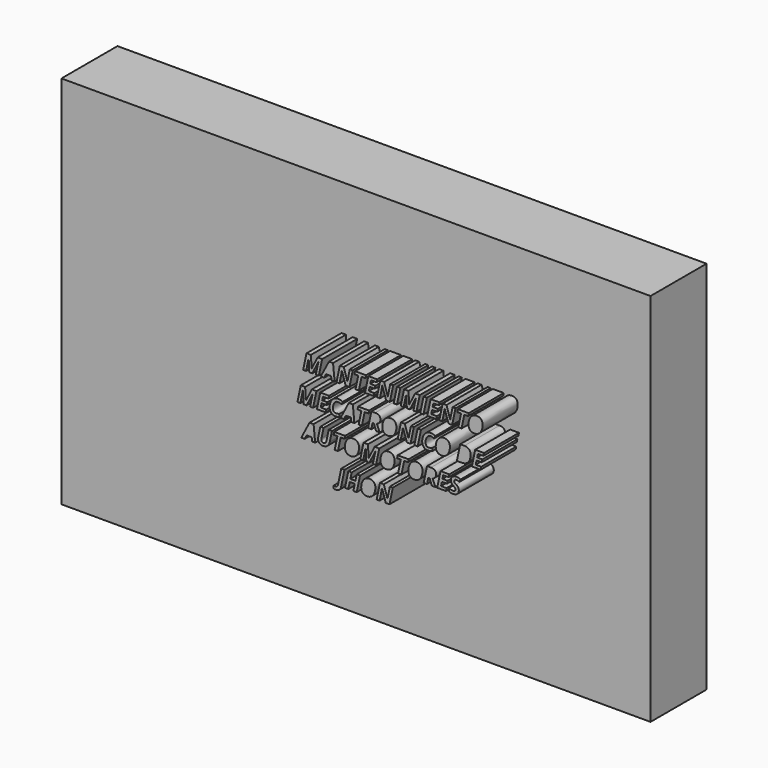
from build123d import *

# Parameters (mm, degrees)
F0_W         = 143.1818306446
F0_H         = 107.0454642177
F1_DEPTH     = 20
F3_DEPTH     = 25
F2_TEXT_SIZE = 6.3131304665
F4_DEPTH     = 12.5


# Not quite as in the source:
# - Text() gives the source's letters only with a copy of the font that has no kerning and outlines rounded to 1/6400 em; it was checked with that copy


with BuildPart() as f1:
    # F0 (on Front) → F1 (new body)
    with BuildSketch(Plane.XZ):
        Rectangle(F0_W, F0_H)
    extrude(amount=F1_DEPTH)

    # F3 (add): a face of the model
    f3_faces = [f1.faces().sort_by_distance(p)[0] for p in [
        (-71.5909153223, -10, 0),
    ]]
    extrude(f3_faces, amount=F3_DEPTH)

    # F2 (on face) → F4 (join, symmetric)
    with BuildSketch(Plane.XZ.offset(20)):
        with Locations((-7.8935887165, -14.7348443667)):
            Text('JHON', F2_TEXT_SIZE, font='Open Sans', font_style=FontStyle.BOLDITALIC, text_align=(TextAlign.LEFT, TextAlign.BOTTOM))
        with Locations((-17.7361536844, -6.1489869323)):
            Text('AUTOMOTORES', F2_TEXT_SIZE, font='Open Sans', font_style=FontStyle.BOLDITALIC, text_align=(TextAlign.LEFT, TextAlign.BOTTOM))
        with BuildLine():
            add(Edge.make_bspline(
                [(7.8744410502, 5.9801149764), (7.6741964432, 6.2188302222), (7.3102050147, 6.2188302222)],
                knots=[0, 0, 0, 1, 1, 1], degree=2))
            add(Edge.make_bspline(
                [(7.3102050147, 6.2188302222), (6.9373357465, 6.2188302222), (6.6261181431, 5.9372054178)],
                knots=[0, 0, 0, 1, 1, 1], degree=2))
            add(Edge.make_bspline(
                [(6.6261181431, 5.9372054178), (6.3149005396, 5.6555806134), (6.1373437452, 5.1623672957)],
                knots=[0, 0, 0, 1, 1, 1], degree=2))
            add(Edge.make_bspline(
                [(6.1373437452, 5.1623672957), (5.9597869509, 4.669153978), (5.9597869509, 4.0920943963)],
                knots=[0, 0, 0, 1, 1, 1], degree=2))
            add(Edge.make_bspline(
                [(5.9597869509, 4.0920943963), (5.9597869509, 3.6393245706), (6.164963691, 3.4080075246)],
                knots=[0, 0, 0, 1, 1, 1], degree=2))
            add(Edge.make_bspline(
                [(6.164963691, 3.4080075246), (6.3701404312, 3.1766904786), (6.7430096994, 3.1766904786)],
                knots=[0, 0, 0, 1, 1, 1], degree=2))
            add(Edge.make_bspline(
                [(6.7430096994, 3.1766904786), (7.1158789675, 3.1766904786), (7.4226576512, 3.4449985235)],
                knots=[0, 0, 0, 1, 1, 1], degree=2))
            add(Edge.make_bspline(
                [(7.4226576512, 3.4449985235), (7.7294363348, 3.7133065683), (7.902060996, 4.2035606061)],
                knots=[0, 0, 0, 1, 1, 1], degree=2))
            add(Edge.make_bspline(
                [(7.902060996, 4.2035606061), (8.0746856571, 4.6938146439), (8.0746856571, 5.3034263045)],
                knots=[0, 0, 0, 1, 1, 1], degree=2))
            add(Edge.make_bspline(
                [(8.0746856571, 5.3034263045), (8.0746856571, 5.7413997306), (7.8744410502, 5.9801149764)],
                knots=[0, 0, 0, 1, 1, 1], degree=2))
        make_face()
        with BuildLine():
            add(Edge.make_bspline(
                [(32.4936770161, 14.5659724108), (32.2934324092, 14.8046876566), (31.9294409807, 14.8046876566)],
                knots=[0, 0, 0, 1, 1, 1], degree=2))
            add(Edge.make_bspline(
                [(31.9294409807, 14.8046876566), (31.5565717125, 14.8046876566), (31.2453541091, 14.5230628522)],
                knots=[0, 0, 0, 1, 1, 1], degree=2))
            add(Edge.make_bspline(
                [(31.2453541091, 14.5230628522), (30.9341365056, 14.2414380478), (30.7565797112, 13.7482247301)],
                knots=[0, 0, 0, 1, 1, 1], degree=2))
            add(Edge.make_bspline(
                [(30.7565797112, 13.7482247301), (30.5790229169, 13.2550114124), (30.5790229169, 12.6779518307)],
                knots=[0, 0, 0, 1, 1, 1], degree=2))
            add(Edge.make_bspline(
                [(30.5790229169, 12.6779518307), (30.5790229169, 12.225182005), (30.784199657, 11.993864959)],
                knots=[0, 0, 0, 1, 1, 1], degree=2))
            add(Edge.make_bspline(
                [(30.784199657, 11.993864959), (30.9893763972, 11.762547913), (31.3622456654, 11.762547913)],
                knots=[0, 0, 0, 1, 1, 1], degree=2))
            add(Edge.make_bspline(
                [(31.3622456654, 11.762547913), (31.7351149335, 11.762547913), (32.0418936171, 12.0308559579)],
                knots=[0, 0, 0, 1, 1, 1], degree=2))
            add(Edge.make_bspline(
                [(32.0418936171, 12.0308559579), (32.3486723007, 12.2991640027), (32.5212969619, 12.7894180405)],
                knots=[0, 0, 0, 1, 1, 1], degree=2))
            add(Edge.make_bspline(
                [(32.5212969619, 12.7894180405), (32.6939216231, 13.2796720783), (32.6939216231, 13.8892837389)],
                knots=[0, 0, 0, 1, 1, 1], degree=2))
            add(Edge.make_bspline(
                [(32.6939216231, 13.8892837389), (32.6939216231, 14.3272571651), (32.4936770161, 14.5659724108)],
                knots=[0, 0, 0, 1, 1, 1], degree=2))
        make_face()
        with BuildLine():
            add(Edge.make_bspline(
                [(15.3160435875, -2.605742458), (15.1157989805, -2.3670272122), (14.7518075521, -2.3670272122)],
                knots=[0, 0, 0, 1, 1, 1], degree=2))
            add(Edge.make_bspline(
                [(14.7518075521, -2.3670272122), (14.3789382839, -2.3670272122), (14.0677206804, -2.6486520166)],
                knots=[0, 0, 0, 1, 1, 1], degree=2))
            add(Edge.make_bspline(
                [(14.0677206804, -2.6486520166), (13.756503077, -2.930276821), (13.5789462826, -3.4234901387)],
                knots=[0, 0, 0, 1, 1, 1], degree=2))
            add(Edge.make_bspline(
                [(13.5789462826, -3.4234901387), (13.4013894882, -3.9167034564), (13.4013894882, -4.4937630381)],
                knots=[0, 0, 0, 1, 1, 1], degree=2))
            add(Edge.make_bspline(
                [(13.4013894882, -4.4937630381), (13.4013894882, -4.9465328638), (13.6065662284, -5.1778499098)],
                knots=[0, 0, 0, 1, 1, 1], degree=2))
            add(Edge.make_bspline(
                [(13.6065662284, -5.1778499098), (13.8117429686, -5.4091669558), (14.1846122367, -5.4091669558)],
                knots=[0, 0, 0, 1, 1, 1], degree=2))
            add(Edge.make_bspline(
                [(14.1846122367, -5.4091669558), (14.5574815049, -5.4091669558), (14.8642601885, -5.1408589109)],
                knots=[0, 0, 0, 1, 1, 1], degree=2))
            add(Edge.make_bspline(
                [(14.8642601885, -5.1408589109), (15.1710388721, -4.8725508661), (15.3436635333, -4.3822968283)],
                knots=[0, 0, 0, 1, 1, 1], degree=2))
            add(Edge.make_bspline(
                [(15.3436635333, -4.3822968283), (15.5162881945, -3.8920427905), (15.5162881945, -3.2824311299)],
                knots=[0, 0, 0, 1, 1, 1], degree=2))
            add(Edge.make_bspline(
                [(15.5162881945, -3.2824311299), (15.5162881945, -2.8444577038), (15.3160435875, -2.605742458)],
                knots=[0, 0, 0, 1, 1, 1], degree=2))
        make_face()
        with BuildLine():
            add(Edge.make_bspline(
                [(7.3565670666, -2.605742458), (7.1563224596, -2.3670272122), (6.7923310311, -2.3670272122)],
                knots=[0, 0, 0, 1, 1, 1], degree=2))
            add(Edge.make_bspline(
                [(6.7923310311, -2.3670272122), (6.419461763, -2.3670272122), (6.1082441595, -2.6486520166)],
                knots=[0, 0, 0, 1, 1, 1], degree=2))
            add(Edge.make_bspline(
                [(6.1082441595, -2.6486520166), (5.797026556, -2.930276821), (5.6194697617, -3.4234901387)],
                knots=[0, 0, 0, 1, 1, 1], degree=2))
            add(Edge.make_bspline(
                [(5.6194697617, -3.4234901387), (5.4419129673, -3.9167034564), (5.4419129673, -4.4937630381)],
                knots=[0, 0, 0, 1, 1, 1], degree=2))
            add(Edge.make_bspline(
                [(5.4419129673, -4.4937630381), (5.4419129673, -4.9465328638), (5.6470897075, -5.1778499098)],
                knots=[0, 0, 0, 1, 1, 1], degree=2))
            add(Edge.make_bspline(
                [(5.6470897075, -5.1778499098), (5.8522664476, -5.4091669558), (6.2251357158, -5.4091669558)],
                knots=[0, 0, 0, 1, 1, 1], degree=2))
            add(Edge.make_bspline(
                [(6.2251357158, -5.4091669558), (6.598004984, -5.4091669558), (6.9047836676, -5.1408589109)],
                knots=[0, 0, 0, 1, 1, 1], degree=2))
            add(Edge.make_bspline(
                [(6.9047836676, -5.1408589109), (7.2115623512, -4.8725508661), (7.3841870124, -4.3822968283)],
                knots=[0, 0, 0, 1, 1, 1], degree=2))
            add(Edge.make_bspline(
                [(7.3841870124, -4.3822968283), (7.5568116736, -3.8920427905), (7.5568116736, -3.2824311299)],
                knots=[0, 0, 0, 1, 1, 1], degree=2))
            add(Edge.make_bspline(
                [(7.5568116736, -3.2824311299), (7.5568116736, -2.8444577038), (7.3565670666, -2.605742458)],
                knots=[0, 0, 0, 1, 1, 1], degree=2))
        make_face()
        with BuildLine():
            add(Edge.make_bspline(
                [(23.1423525127, 5.9801149764), (22.9421079057, 6.2188302222), (22.5781164772, 6.2188302222)],
                knots=[0, 0, 0, 1, 1, 1], degree=2))
            add(Edge.make_bspline(
                [(22.5781164772, 6.2188302222), (22.2052472091, 6.2188302222), (21.8940296056, 5.9372054178)],
                knots=[0, 0, 0, 1, 1, 1], degree=2))
            add(Edge.make_bspline(
                [(21.8940296056, 5.9372054178), (21.5828120021, 5.6555806134), (21.4052552078, 5.1623672957)],
                knots=[0, 0, 0, 1, 1, 1], degree=2))
            add(Edge.make_bspline(
                [(21.4052552078, 5.1623672957), (21.2276984134, 4.669153978), (21.2276984134, 4.0920943963)],
                knots=[0, 0, 0, 1, 1, 1], degree=2))
            add(Edge.make_bspline(
                [(21.2276984134, 4.0920943963), (21.2276984134, 3.6393245706), (21.4328751536, 3.4080075246)],
                knots=[0, 0, 0, 1, 1, 1], degree=2))
            add(Edge.make_bspline(
                [(21.4328751536, 3.4080075246), (21.6380518937, 3.1766904786), (22.0109211619, 3.1766904786)],
                knots=[0, 0, 0, 1, 1, 1], degree=2))
            add(Edge.make_bspline(
                [(22.0109211619, 3.1766904786), (22.3837904301, 3.1766904786), (22.6905691137, 3.4449985235)],
                knots=[0, 0, 0, 1, 1, 1], degree=2))
            add(Edge.make_bspline(
                [(22.6905691137, 3.4449985235), (22.9973477973, 3.7133065683), (23.1699724585, 4.2035606061)],
                knots=[0, 0, 0, 1, 1, 1], degree=2))
            add(Edge.make_bspline(
                [(23.1699724585, 4.2035606061), (23.3425971197, 4.6938146439), (23.3425971197, 5.3034263045)],
                knots=[0, 0, 0, 1, 1, 1], degree=2))
            add(Edge.make_bspline(
                [(23.3425971197, 5.3034263045), (23.3425971197, 5.7413997306), (23.1423525127, 5.9801149764)],
                knots=[0, 0, 0, 1, 1, 1], degree=2))
        make_face()
        with BuildLine():
            add(Edge.make_bspline(
                [(1.8690756939, -11.1915998924), (1.6688310869, -10.9528846466), (1.3048396585, -10.9528846466)],
                knots=[0, 0, 0, 1, 1, 1], degree=2))
            add(Edge.make_bspline(
                [(1.3048396585, -10.9528846466), (0.9319703903, -10.9528846466), (0.6207527868, -11.234509451)],
                knots=[0, 0, 0, 1, 1, 1], degree=2))
            add(Edge.make_bspline(
                [(0.6207527868, -11.234509451), (0.3095351834, -11.5161342554), (0.131978389, -12.0093475731)],
                knots=[0, 0, 0, 1, 1, 1], degree=2))
            add(Edge.make_bspline(
                [(0.131978389, -12.0093475731), (-0.0455784054, -12.5025608908), (-0.0455784054, -13.0796204725)],
                knots=[0, 0, 0, 1, 1, 1], degree=2))
            add(Edge.make_bspline(
                [(-0.0455784054, -13.0796204725), (-0.0455784054, -13.5323902982), (0.1595983348, -13.7637073442)],
                knots=[0, 0, 0, 1, 1, 1], degree=2))
            add(Edge.make_bspline(
                [(0.1595983348, -13.7637073442), (0.364775075, -13.9950243902), (0.7376443431, -13.9950243902)],
                knots=[0, 0, 0, 1, 1, 1], degree=2))
            add(Edge.make_bspline(
                [(0.7376443431, -13.9950243902), (1.1105136113, -13.9950243902), (1.4172922949, -13.7267163453)],
                knots=[0, 0, 0, 1, 1, 1], degree=2))
            add(Edge.make_bspline(
                [(1.4172922949, -13.7267163453), (1.7240709785, -13.4584083005), (1.8966956397, -12.9681542627)],
                knots=[0, 0, 0, 1, 1, 1], degree=2))
            add(Edge.make_bspline(
                [(1.8966956397, -12.9681542627), (2.0693203009, -12.4779002249), (2.0693203009, -11.8682885643)],
                knots=[0, 0, 0, 1, 1, 1], degree=2))
            add(Edge.make_bspline(
                [(2.0693203009, -11.8682885643), (2.0693203009, -11.4303151382), (1.8690756939, -11.1915998924)],
                knots=[0, 0, 0, 1, 1, 1], degree=2))
        make_face()
        with BuildLine():
            add(Edge.make_bspline(
                [(-2.8065865578, -2.605742458), (-3.0068311648, -2.3670272122), (-3.3708225932, -2.3670272122)],
                knots=[0, 0, 0, 1, 1, 1], degree=2))
            add(Edge.make_bspline(
                [(-3.3708225932, -2.3670272122), (-3.7436918614, -2.3670272122), (-4.0549094649, -2.6486520166)],
                knots=[0, 0, 0, 1, 1, 1], degree=2))
            add(Edge.make_bspline(
                [(-4.0549094649, -2.6486520166), (-4.3661270684, -2.930276821), (-4.5436838627, -3.4234901387)],
                knots=[0, 0, 0, 1, 1, 1], degree=2))
            add(Edge.make_bspline(
                [(-4.5436838627, -3.4234901387), (-4.7212406571, -3.9167034564), (-4.7212406571, -4.4937630381)],
                knots=[0, 0, 0, 1, 1, 1], degree=2))
            add(Edge.make_bspline(
                [(-4.7212406571, -4.4937630381), (-4.7212406571, -4.9465328638), (-4.5160639169, -5.1778499098)],
                knots=[0, 0, 0, 1, 1, 1], degree=2))
            add(Edge.make_bspline(
                [(-4.5160639169, -5.1778499098), (-4.3108871768, -5.4091669558), (-3.9380179086, -5.4091669558)],
                knots=[0, 0, 0, 1, 1, 1], degree=2))
            add(Edge.make_bspline(
                [(-3.9380179086, -5.4091669558), (-3.5651486404, -5.4091669558), (-3.2583699568, -5.1408589109)],
                knots=[0, 0, 0, 1, 1, 1], degree=2))
            add(Edge.make_bspline(
                [(-3.2583699568, -5.1408589109), (-2.9515912732, -4.8725508661), (-2.778966612, -4.3822968283)],
                knots=[0, 0, 0, 1, 1, 1], degree=2))
            add(Edge.make_bspline(
                [(-2.778966612, -4.3822968283), (-2.6063419508, -3.8920427905), (-2.6063419508, -3.2824311299)],
                knots=[0, 0, 0, 1, 1, 1], degree=2))
            add(Edge.make_bspline(
                [(-2.6063419508, -3.2824311299), (-2.6063419508, -2.8444577038), (-2.8065865578, -2.605742458)],
                knots=[0, 0, 0, 1, 1, 1], degree=2))
        make_face()
        with Locations((-17.7361536844, 11.0227279365)):
            Text('MANTENIMIENTO', F2_TEXT_SIZE, font='Open Sans', font_style=FontStyle.BOLDITALIC, text_align=(TextAlign.LEFT, TextAlign.BOTTOM))
        with Locations((-19.376581179, 2.4368705021)):
            Text('MECATRONICO DE', F2_TEXT_SIZE, font='Open Sans', font_style=FontStyle.BOLDITALIC, text_align=(TextAlign.LEFT, TextAlign.BOTTOM))
        with BuildLine():
            Line((27.4096341374, 3.2260118104), (27.7361413537, 3.2260118104))
            add(Edge.make_bspline(
                [(27.7361413537, 3.2260118104), (28.1918704592, 3.2260118104), (28.5312012218, 3.4602881363)],
                knots=[0, 0, 0, 1, 1, 1], degree=2))
            add(Edge.make_bspline(
                [(28.5312012218, 3.4602881363), (28.8705319844, 3.6945644622), (29.0614055383, 4.1493071411)],
                knots=[0, 0, 0, 1, 1, 1], degree=2))
            add(Edge.make_bspline(
                [(29.0614055383, 4.1493071411), (29.2522790923, 4.60404982), (29.2522790923, 5.1899872415)],
                knots=[0, 0, 0, 1, 1, 1], degree=2))
            add(Edge.make_bspline(
                [(29.2522790923, 5.1899872415), (29.2522790923, 5.6644584531), (29.0288534593, 5.9125447519)],
                knots=[0, 0, 0, 1, 1, 1], degree=2))
            add(Edge.make_bspline(
                [(29.0288534593, 5.9125447519), (28.8054278264, 6.1606310507), (28.3861965064, 6.1606310507)],
                knots=[0, 0, 0, 1, 1, 1], degree=2))
            Line((28.3861965064, 6.1606310507), (28.0320693443, 6.1606310507))
            Line((28.0320693443, 6.1606310507), (27.4096341374, 3.2260118104))
        make_face()
        with BuildLine():
            Line((18.5653329245, -2.4252263837), (18.3059027194, -3.6424768518))
            Line((18.3059027194, -3.6424768518), (18.5465908184, -3.6424768518))
            add(Edge.make_bspline(
                [(18.5465908184, -3.6424768518), (18.9500393123, -3.6424768518), (19.1754377985, -3.4668929107)],
                knots=[0, 0, 0, 1, 1, 1], degree=2))
            add(Edge.make_bspline(
                [(19.1754377985, -3.4668929107), (19.4008362847, -3.2913089696), (19.4008362847, -2.930276821)],
                knots=[0, 0, 0, 1, 1, 1], degree=2))
            add(Edge.make_bspline(
                [(19.4008362847, -2.930276821), (19.4008362847, -2.6777516024), (19.2543519293, -2.551488993)],
                knots=[0, 0, 0, 1, 1, 1], degree=2))
            add(Edge.make_bspline(
                [(19.2543519293, -2.551488993), (19.1078675739, -2.4252263837), (18.7931974773, -2.4252263837)],
                knots=[0, 0, 0, 1, 1, 1], degree=2))
            Line((18.7931974773, -2.4252263837), (18.5653329245, -2.4252263837))
        make_face()
        with BuildLine():
            Line((2.6710405485, 6.1606310507), (2.4116103434, 4.9433805826))
            Line((2.4116103434, 4.9433805826), (2.6522984424, 4.9433805826))
            add(Edge.make_bspline(
                [(2.6522984424, 4.9433805826), (3.0557469363, 4.9433805826), (3.2811454225, 5.1189645237)],
                knots=[0, 0, 0, 1, 1, 1], degree=2))
            add(Edge.make_bspline(
                [(3.2811454225, 5.1189645237), (3.5065439087, 5.2945484648), (3.5065439087, 5.6555806134)],
                knots=[0, 0, 0, 1, 1, 1], degree=2))
            add(Edge.make_bspline(
                [(3.5065439087, 5.6555806134), (3.5065439087, 5.908105832), (3.3600595533, 6.0343684414)],
                knots=[0, 0, 0, 1, 1, 1], degree=2))
            add(Edge.make_bspline(
                [(3.3600595533, 6.0343684414), (3.213575198, 6.1606310507), (2.8989051013, 6.1606310507)],
                knots=[0, 0, 0, 1, 1, 1], degree=2))
            Line((2.8989051013, 6.1606310507), (2.6710405485, 6.1606310507))
        make_face()
        with BuildLine():
            Line((-16.2131109593, -4.2747763251), (-15.1872272585, -4.2747763251))
            Line((-15.1872272585, -4.2747763251), (-15.267127816, -3.195625586))
            add(Edge.make_bspline(
                [(-15.267127816, -3.195625586), (-15.2977070417, -2.7921770921), (-15.2977070417, -2.416348544)],
                knots=[0, 0, 0, 1, 1, 1], degree=2))
            Line((-15.2977070417, -2.416348544), (-15.2977070417, -2.3048823342))
            add(Edge.make_bspline(
                [(-15.2977070417, -2.3048823342), (-15.4338339174, -2.6747923225), (-15.6340785244, -3.0881050827)],
                knots=[0, 0, 0, 1, 1, 1], degree=2))
            Line((-15.6340785244, -3.0881050827), (-16.2131109593, -4.2747763251))
        make_face()
        with BuildLine():
            Line((-10.6585425755, 12.8969385437), (-9.6326588747, 12.8969385437))
            Line((-9.6326588747, 12.8969385437), (-9.7125594321, 13.9760892829))
            add(Edge.make_bspline(
                [(-9.7125594321, 13.9760892829), (-9.7431386578, 14.3795377767), (-9.7431386578, 14.7553663248)],
                knots=[0, 0, 0, 1, 1, 1], degree=2))
            Line((-9.7431386578, 14.7553663248), (-9.7431386578, 14.8668325346))
            add(Edge.make_bspline(
                [(-9.7431386578, 14.8668325346), (-9.8792655335, 14.4969225463), (-10.0795101405, 14.0836097861)],
                knots=[0, 0, 0, 1, 1, 1], degree=2))
            Line((-10.0795101405, 14.0836097861), (-10.6585425755, 12.8969385437))
        make_face()
        with BuildLine():
            Line((-5.0142093678, 4.3110811093), (-3.988325667, 4.3110811093))
            Line((-3.988325667, 4.3110811093), (-4.0682262245, 5.3902318484))
            add(Edge.make_bspline(
                [(-4.0682262245, 5.3902318484), (-4.0988054502, 5.7936803423), (-4.0988054502, 6.1695088904)],
                knots=[0, 0, 0, 1, 1, 1], degree=2))
            Line((-4.0988054502, 6.1695088904), (-4.0988054502, 6.2809751002))
            add(Edge.make_bspline(
                [(-4.0988054502, 6.2809751002), (-4.2349323258, 5.9110651119), (-4.4351769328, 5.4977523517)],
                knots=[0, 0, 0, 1, 1, 1], degree=2))
            Line((-4.4351769328, 5.4977523517), (-5.0142093678, 4.3110811093))
        make_face()
    extrude(amount=F4_DEPTH, both=True)


solid = f1.part
